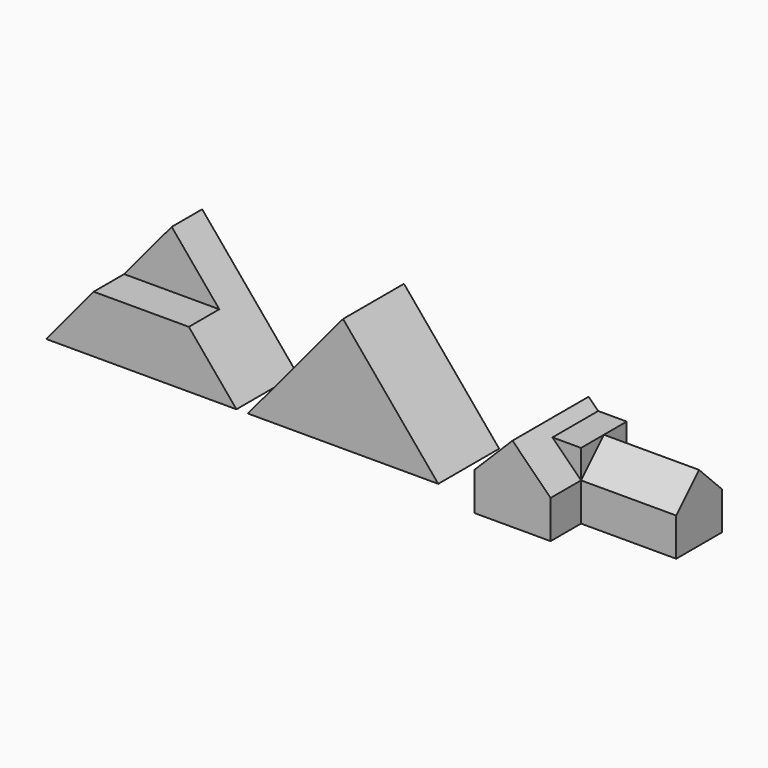
from build123d import *

# Parameters (mm, degrees)
F1_DEPTH  = 101.6
F3_DEPTH  = 50.8
F5_DEPTH  = 101.6
F7_DEPTH  = 127
F6_W      = 127
F6_H      = 50.8
F8_DEPTH  = 76.2
F9_DEPTH  = 76.2
F11_DEPTH = 127
F13_DEPTH = 127


with BuildPart() as f1:
    # F0 (on Front) → F1 (new body)
    with BuildSketch(Plane.XZ):
        Polygon((127, 152.4), (0, 0), (254, 0), align=None)
    extrude(amount=F1_DEPTH)

    # F2 (on face) → F3 (cut)
    with BuildSketch(Plane.XZ.offset(101.6)):
        Polygon((63.5, 76.2), (127, 76.2), (190.5, 76.2), (127, 152.4), align=None)
    extrude(amount=-F3_DEPTH, mode=Mode.SUBTRACT)


with BuildPart() as f5:
    # F4 (on Front) → F5 (new body)
    with BuildSketch(Plane.XZ):
        Polygon((396.2579253727, 152.4), (269.2579253727, 0), (523.2579253727, 0), align=None)
    extrude(amount=F5_DEPTH)


with BuildPart() as f7:
    # F6 (on Front) → F7 (new body)
    with BuildSketch(Plane.XZ):
        Polygon((591.8814198494, 49.1360899748), (591.8814198494, -1.6639100252), (693.4814198494, -1.6639100252), (693.4814198494, 49.1360899748), (655.3814198494, 87.2360899748), (642.6814198494, 99.9360899748), align=None)
    extrude(amount=F7_DEPTH)

    # F6 (on Front) → F8 (join)
    with BuildSketch(Plane.XZ):
        with Locations((756.9814198494, 23.7360899748)):
            Rectangle(F6_W, F6_H)
    extrude(amount=F8_DEPTH)

    # F6 (on Front) → F9 (join)
    with BuildSketch(Plane.XZ):
        Polygon((655.3814198494, 87.2360899748), (693.4814198494, 49.1360899748), (820.4814198494, 49.1360899748), (820.4814198494, 87.2360899748), align=None)
    extrude(amount=F9_DEPTH)

    # F10 (on face) → F11 (cut)
    with BuildSketch(Plane.YZ.offset(820.4814198494)):
        Polygon((-76.2, 87.2360899748), (-76.2, 49.1362325847), (-38.1, 87.2360899748), align=None)
    extrude(amount=-F11_DEPTH, mode=Mode.SUBTRACT)

    # F12 (on face) → F13 (cut)
    with BuildSketch(Plane.YZ.offset(820.4814198494)):
        Polygon((0, 87.2360899748), (-38.1, 87.2360899748), (0, 49.1362325847), align=None)
    extrude(amount=-F13_DEPTH, mode=Mode.SUBTRACT)


solid = Compound([f1.part, f5.part, f7.part])
